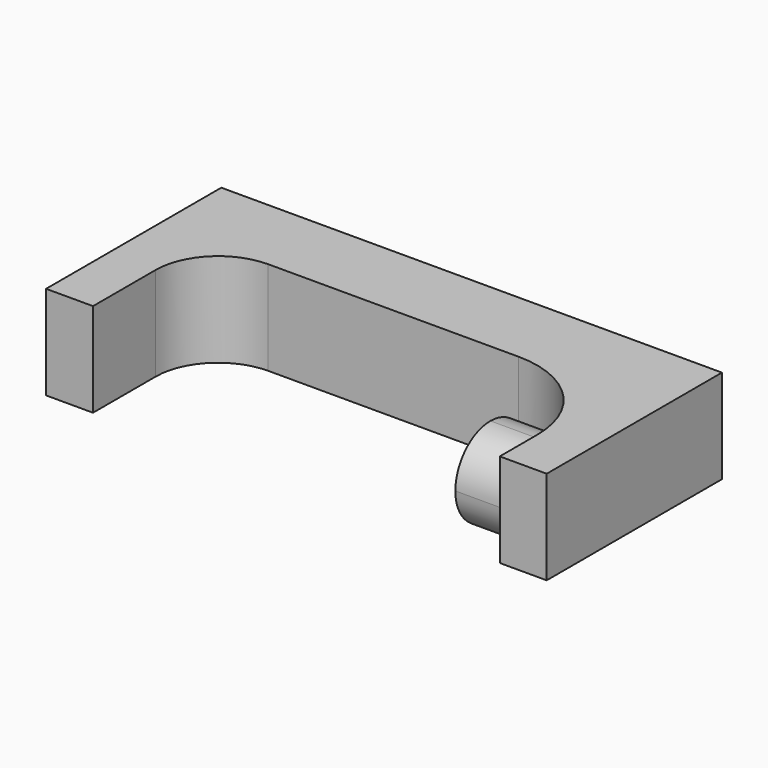
from build123d import *

# Parameters (mm, degrees)
F1_DEPTH = 3
F2_R     = 3
F3_R     = 2
F5_DEPTH = 1.5


with BuildPart() as f1:
    # F0 (on Top) → F1 (new body)
    with BuildSketch(Plane.XY):
        Polygon((-3.2379887671, -1), (-1.7379887671, -1), (-1.7379887671, 3.5), (11.2620112329, 3.5), (11.2620112329, -1), (12.7620112329, -1), (12.7620112329, 6), (-3.2379887671, 6), align=None)
    extrude(amount=F1_DEPTH)

    # F2
    f2_edges = [f1.edges().sort_by_distance(p)[0] for p in [
        (11.262011, 3.5, 1.5),
    ]]
    fillet(f2_edges, radius=F2_R)

    # F3
    f3_edges = [f1.edges().sort_by_distance(p)[0] for p in [
        (-1.737989, 3.5, 1.5),
    ]]
    fillet(f3_edges, radius=F3_R)


with BuildPart() as f5:
    # F4 (on face) → F5 (new body)
    with BuildSketch(Plane(origin=(11.2620112329, 0, 0), x_dir=(0, -1, 0), z_dir=(-1, 0, 0))):
        with BuildLine():
            ThreePointArc((-0.5, 0.1), (0.4899494937, 0.5100505063), (0.9, 1.5))
            ThreePointArc((0.9, 1.5), (0.4899494937, 2.4899494937), (-0.5, 2.9))
            Line((-0.5, 2.9), (-0.5, 0.1))
        make_face()
        with BuildLine():
            Line((-0.5, 0.1), (-0.5, 2.9))
            ThreePointArc((-0.5, 2.9), (-1.9, 1.5), (-0.5, 0.1))
        make_face()
    extrude(amount=F5_DEPTH)


solid = Compound([f1.part, f5.part])
